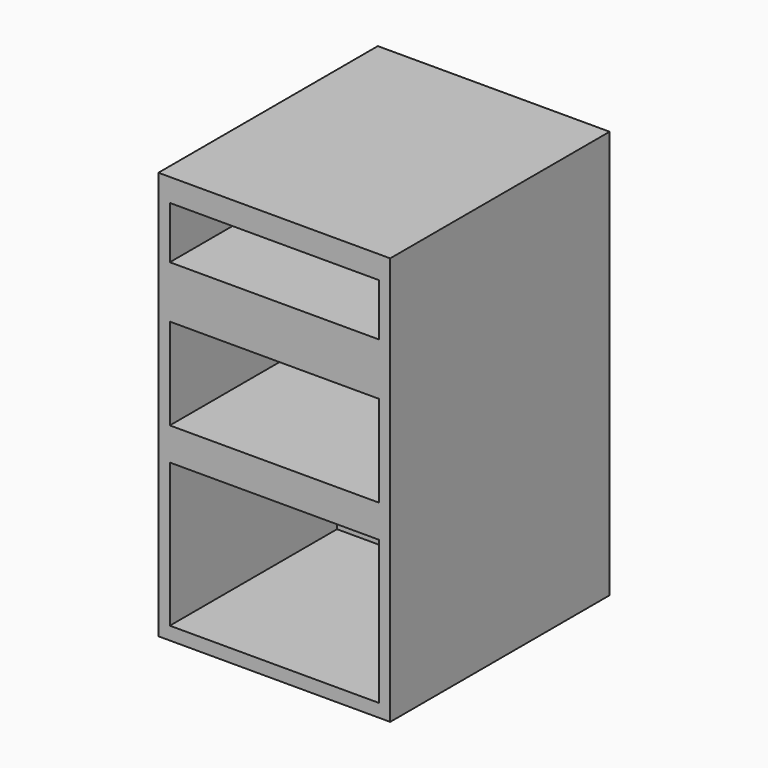
from build123d import *

# Parameters (mm, degrees)
F0_W     = 450.85
F0_H     = 533.4
F1_DEPTH = 793.75
F2_W     = 406.4
F2_H     = 101.6
F2_H_2   = 177.8
F2_H_3   = 279.4
F3_DEPTH = 406.4


# Not quite as in the source:
# - a feature names something its author has since deleted; it is built from what else it names


with BuildPart() as f1:
    # F0 (on Top) → F1 (new body)
    with BuildSketch(Plane.XY):
        Rectangle(F0_W, F0_H)
    extrude(amount=-F1_DEPTH)

    # F2 (on face) → F3 (cut)
    with BuildSketch(Plane.XZ.offset(266.7)):
        with Locations((0, -95.25)):
            Rectangle(F2_W, F2_H)
        with Locations((0, -336.55)):
            Rectangle(F2_W, F2_H_2)
        with Locations((0, -628.65)):
            Rectangle(F2_W, F2_H_3)
    extrude(amount=-F3_DEPTH, mode=Mode.SUBTRACT)


solid = f1.part
